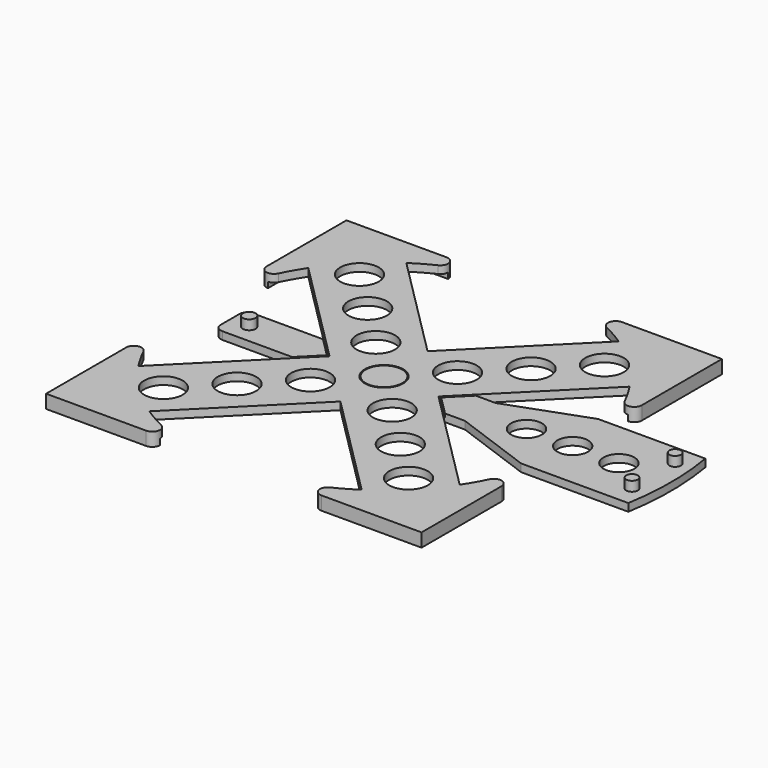
from build123d import *

# Parameters (mm, degrees)
F0_R           = 5
F1_DEPTH       = 2
F3_DEPTH       = 1.5
F4_R           = 1.5
F5_DEPTH       = 2.5
F7_W           = 65
F7_H           = 10
F7_R           = 4
F8_DEPTH       = 2
F9_R           = 1.65
F9_R_2         = 1.5
F10_DEPTH      = 2.5
F11_R          = 4.75
F12_DEPTH      = 1
F13_DEPTH      = 1
F14_T1_DEPTH   = 61.7948981324
F14_2_T1_DEPTH = 12


# Not quite as in the source:
# - a fillet or chamfer that OpenCascade refuses, or shapes differently, is made with other operations: its cross-section is extruded or revolved along the edge and cut away or added


with BuildPart() as f1:
    # F0 (on Top) → F1 (new body)
    with BuildSketch(Plane.XY):
        with BuildLine():
            Line((-11.1102430216, 48.75), (-48.75, 48.75))
            Line((-48.75, 48.75), (-48.75, 11.1102430216))
            ThreePointArc((-48.75, 11.1102430216), (-45.9736623898, 19.6576287092), (-41.7120839632, 27.5699483395))
            Line((-41.7120839632, 27.5699483395), (-14.1421356237, 0))
            Line((-14.1421356237, 0), (-41.7120839632, -27.5699483395))
            ThreePointArc((-41.7120839632, -27.5699483395), (-45.9736623898, -19.6576287092), (-48.75, -11.1102430216))
            Line((-48.75, -11.1102430216), (-48.75, -48.75))
            Line((-48.75, -48.75), (-11.1102430216, -48.75))
            ThreePointArc((-11.1102430216, -48.75), (-19.6576287092, -45.9736623898), (-27.5699483395, -41.7120839632))
            Line((-27.5699483395, -41.7120839632), (0, -14.1421356237))
            Line((0, -14.1421356237), (27.5699483395, -41.7120839632))
            ThreePointArc((27.5699483395, -41.7120839632), (19.6576287092, -45.9736623898), (11.1102430216, -48.75))
            Line((11.1102430216, -48.75), (48.75, -48.75))
            Line((48.75, -48.75), (48.75, -11.1102430216))
            ThreePointArc((48.75, -11.1102430216), (45.9736623898, -19.6576287092), (41.7120839632, -27.5699483395))
            Line((41.7120839632, -27.5699483395), (14.1421356237, 0))
            Line((14.1421356237, 0), (41.7120839632, 27.5699483395))
            ThreePointArc((41.7120839632, 27.5699483395), (45.9736623898, 19.6576287092), (48.75, 11.1102430216))
            Line((48.75, 11.1102430216), (48.75, 48.75))
            Line((48.75, 48.75), (11.1102430216, 48.75))
            ThreePointArc((11.1102430216, 48.75), (19.6576287092, 45.9736623898), (27.5699483395, 41.7120839632))
            Line((27.5699483395, 41.7120839632), (0, 14.1421356237))
            Line((0, 14.1421356237), (-27.5699483395, 41.7120839632))
            ThreePointArc((-27.5699483395, 41.7120839632), (-19.6576287092, 45.9736623898), (-11.1102430216, 48.75))
        make_face()
        with Locations((-31.8198051534, -31.8198051534)):
            Circle(F0_R, mode=Mode.SUBTRACT)
        with Locations((-21.2132034356, -21.2132034356)):
            Circle(F0_R, mode=Mode.SUBTRACT)
        with Locations((-10.6066017178, -10.6066017178)):
            Circle(F0_R, mode=Mode.SUBTRACT)
        with Locations((31.8198051534, -31.8198051534)):
            Circle(F0_R, mode=Mode.SUBTRACT)
        with Locations((21.2132034356, -21.2132034356)):
            Circle(F0_R, mode=Mode.SUBTRACT)
        with Locations((10.6066017178, -10.6066017178)):
            Circle(F0_R, mode=Mode.SUBTRACT)
        Circle(F0_R, mode=Mode.SUBTRACT)
        with Locations((-10.6066017178, 10.6066017178)):
            Circle(F0_R, mode=Mode.SUBTRACT)
        with Locations((-21.2132034356, 21.2132034356)):
            Circle(F0_R, mode=Mode.SUBTRACT)
        with Locations((-31.8198051534, 31.8198051534)):
            Circle(F0_R, mode=Mode.SUBTRACT)
        with Locations((10.6066017178, 10.6066017178)):
            Circle(F0_R, mode=Mode.SUBTRACT)
        with Locations((21.2132034356, 21.2132034356)):
            Circle(F0_R, mode=Mode.SUBTRACT)
        with Locations((31.8198051534, 31.8198051534)):
            Circle(F0_R, mode=Mode.SUBTRACT)
    extrude(amount=F1_DEPTH)

    # F2 (on face) → F3 (join)
    with BuildSketch(Plane(origin=(0, 0, 0), x_dir=(1, 0, 0), z_dir=(0, 0, -1))):
        with BuildLine():
            Line((46.75, -46.75), (17.7323856263, -46.75))
            ThreePointArc((17.7323856263, -46.75), (14.4559436507, -47.8646601698), (11.1102430216, -48.75))
            Line((11.1102430216, -48.75), (48.75, -48.75))
            Line((48.75, -48.75), (48.75, -11.1102430216))
            ThreePointArc((48.75, -11.1102430216), (47.8646601698, -14.4559436507), (46.75, -17.7323856263))
            Line((46.75, -17.7323856263), (46.75, -46.75))
        make_face()
        with BuildLine():
            ThreePointArc((11.1102430216, 48.75), (14.4559436507, 47.8646601698), (17.7323856263, 46.75))
            Line((17.7323856263, 46.75), (46.75, 46.75))
            Line((46.75, 46.75), (46.75, 17.7323856263))
            ThreePointArc((46.75, 17.7323856263), (47.8646601698, 14.4559436507), (48.75, 11.1102430216))
            Line((48.75, 11.1102430216), (48.75, 48.75))
            Line((48.75, 48.75), (11.1102430216, 48.75))
        make_face()
        with BuildLine():
            Line((-17.7323856263, -46.75), (-46.75, -46.75))
            Line((-46.75, -46.75), (-46.75, -17.7323856263))
            ThreePointArc((-46.75, -17.7323856263), (-47.8646601698, -14.4559436507), (-48.75, -11.1102430216))
            Line((-48.75, -11.1102430216), (-48.75, -48.75))
            Line((-48.75, -48.75), (-11.1102430216, -48.75))
            ThreePointArc((-11.1102430216, -48.75), (-14.4559436507, -47.8646601698), (-17.7323856263, -46.75))
        make_face()
        with BuildLine():
            Line((-11.1102430216, 48.75), (-48.75, 48.75))
            Line((-48.75, 48.75), (-48.75, 11.1102430216))
            ThreePointArc((-48.75, 11.1102430216), (-47.8646601698, 14.4559436507), (-46.75, 17.7323856263))
            Line((-46.75, 17.7323856263), (-46.75, 46.75))
            Line((-46.75, 46.75), (-17.7323856263, 46.75))
            ThreePointArc((-17.7323856263, 46.75), (-14.4559436507, 47.8646601698), (-11.1102430216, 48.75))
        make_face()
    extrude(amount=F3_DEPTH)

    # F4 (on face) → F5 (join)
    with BuildSketch(Plane(origin=(0, 0, 0), x_dir=(1, 0, 0), z_dir=(0, 0, -1))):
        with Locations((-40.25, 40.25)):
            Circle(F4_R)
        with Locations((40.25, 40.25)):
            Circle(F4_R)
        with Locations((40.25, -40.25)):
            Circle(F4_R)
        with Locations((-40.25, -40.25)):
            Circle(F4_R)
    extrude(amount=F5_DEPTH)

    # F11 (on offset) → F13 (cut)
    with BuildSketch(Plane.XY.offset(1)):
        Polygon((20.3492424049, -5.5), (14.8492424049, 0), (20.3492424049, 5.5), (-20.3492424049, 5.5), (-14.8492424049, 0), (-20.3492424049, -5.5), align=None)
        Circle(F11_R, mode=Mode.SUBTRACT)
    extrude(amount=-F13_DEPTH, mode=Mode.SUBTRACT)

    # F14: fillet of radius 2 on 8 edges, made by hand

    # F14_s2 → F14_t1 (cut)
    with BuildSketch(Plane.XY.offset(-30.6474490662)):
        with BuildLine():
            ThreePointArc((-48.75, 22.7692226481), (-47.1993585171, 20.8203571004), (-44.9519230769, 21.8934833155))
            ThreePointArc((-44.9519230769, 21.8934833155), (-47.160175624, 16.6107746693), (-48.75, 11.1102430216))
            Line((-48.75, 11.1102430216), (-48.75, 22.7692226481))
        make_face()
        with BuildLine():
            ThreePointArc((-21.8934833155, 44.9519230769), (-20.8203571004, 47.1993585171), (-22.7692226481, 48.75))
            Line((-22.7692226481, 48.75), (-11.1102430216, 48.75))
            ThreePointArc((-11.1102430216, 48.75), (-16.6107746693, 47.160175624), (-21.8934833155, 44.9519230769))
        make_face()
        with BuildLine():
            ThreePointArc((21.8934833155, 44.9519230769), (20.8203571004, 47.1993585171), (22.7692226481, 48.75))
            Line((22.7692226481, 48.75), (11.1102430216, 48.75))
            ThreePointArc((11.1102430216, 48.75), (16.6107746693, 47.160175624), (21.8934833155, 44.9519230769))
        make_face()
        with BuildLine():
            ThreePointArc((48.75, 22.7692226481), (47.1993585171, 20.8203571004), (44.9519230769, 21.8934833155))
            ThreePointArc((44.9519230769, 21.8934833155), (47.160175624, 16.6107746693), (48.75, 11.1102430216))
            Line((48.75, 11.1102430216), (48.75, 22.7692226481))
        make_face()
        with BuildLine():
            ThreePointArc((48.75, -22.7692226481), (47.1993585171, -20.8203571004), (44.9519230769, -21.8934833155))
            ThreePointArc((44.9519230769, -21.8934833155), (47.160175624, -16.6107746693), (48.75, -11.1102430216))
            Line((48.75, -11.1102430216), (48.75, -22.7692226481))
        make_face()
        with BuildLine():
            ThreePointArc((-44.9519230769, -21.8934833155), (-47.1993585171, -20.8203571004), (-48.75, -22.7692226481))
            Line((-48.75, -22.7692226481), (-48.75, -11.1102430216))
            ThreePointArc((-48.75, -11.1102430216), (-47.160175624, -16.6107746693), (-44.9519230769, -21.8934833155))
        make_face()
        with BuildLine():
            ThreePointArc((-22.7692226481, -48.75), (-20.8203571004, -47.1993585171), (-21.8934833155, -44.9519230769))
            ThreePointArc((-21.8934833155, -44.9519230769), (-16.6107746693, -47.160175624), (-11.1102430216, -48.75))
            Line((-11.1102430216, -48.75), (-22.7692226481, -48.75))
        make_face()
        with BuildLine():
            ThreePointArc((21.8934833155, -44.9519230769), (20.8203571004, -47.1993585171), (22.7692226481, -48.75))
            Line((22.7692226481, -48.75), (11.1102430216, -48.75))
            ThreePointArc((11.1102430216, -48.75), (16.6107746693, -47.160175624), (21.8934833155, -44.9519230769))
        make_face()
    extrude(amount=F14_T1_DEPTH, mode=Mode.SUBTRACT)


with BuildPart() as f8:
    # F7 (on Top) → F8 (new body)
    with BuildSketch(Plane.XY):
        with Locations((-7.5, 0)):
            Rectangle(F7_W, F7_H)
        with BuildLine():
            Line((45.6060806459, 12.5), (25, 5))
            Line((25, 5), (25, -5))
            Line((25, -5), (45.6060806459, -12.5))
            Line((45.6060806459, -12.5), (73.4438561079, -12.5))
            ThreePointArc((73.4438561079, -12.5), (74.5, 0), (73.4438561079, 12.5))
            Line((73.4438561079, 12.5), (45.6060806459, 12.5))
        make_face()
        with Locations((37, 0)):
            Circle(F7_R, mode=Mode.SUBTRACT)
        with Locations((49, 0)):
            Circle(F7_R, mode=Mode.SUBTRACT)
        with Locations((61, 0)):
            Circle(F7_R, mode=Mode.SUBTRACT)
    extrude(amount=F8_DEPTH)

    # F9 (on face) → F10 (join)
    with BuildSketch(Plane.XY.offset(2)):
        with Locations((-35, 0)):
            Circle(F9_R)
        with Locations((70, 7)):
            Circle(F9_R_2)
        with Locations((70, -7)):
            Circle(F9_R_2)
    extrude(amount=F10_DEPTH)

    # F11 (on offset) → F12 (cut)
    with BuildSketch(Plane.XY.offset(1)):
        Polygon((20.3492424049, -5.5), (14.8492424049, 0), (20.3492424049, 5.5), (-20.3492424049, 5.5), (-14.8492424049, 0), (-20.3492424049, -5.5), align=None)
        Circle(F11_R, mode=Mode.SUBTRACT)
    extrude(amount=F12_DEPTH, mode=Mode.SUBTRACT)

    # F14#2: fillet of radius 2 on 2 edges, made by hand

    # F14_2_s2 → F14_2_t1 (cut)
    with BuildSketch(Plane.XY.offset(-5)):
        with BuildLine():
            ThreePointArc((-38, 5), (-39.4142135624, 4.4142135624), (-40, 3))
            Line((-40, 3), (-40, 5))
            Line((-40, 5), (-38, 5))
        make_face()
        with BuildLine():
            ThreePointArc((-40, -3), (-39.4142135624, -4.4142135624), (-38, -5))
            Line((-38, -5), (-40, -5))
            Line((-40, -5), (-40, -3))
        make_face()
    extrude(amount=F14_2_T1_DEPTH, mode=Mode.SUBTRACT)


solid = Compound([f1.part, f8.part])
